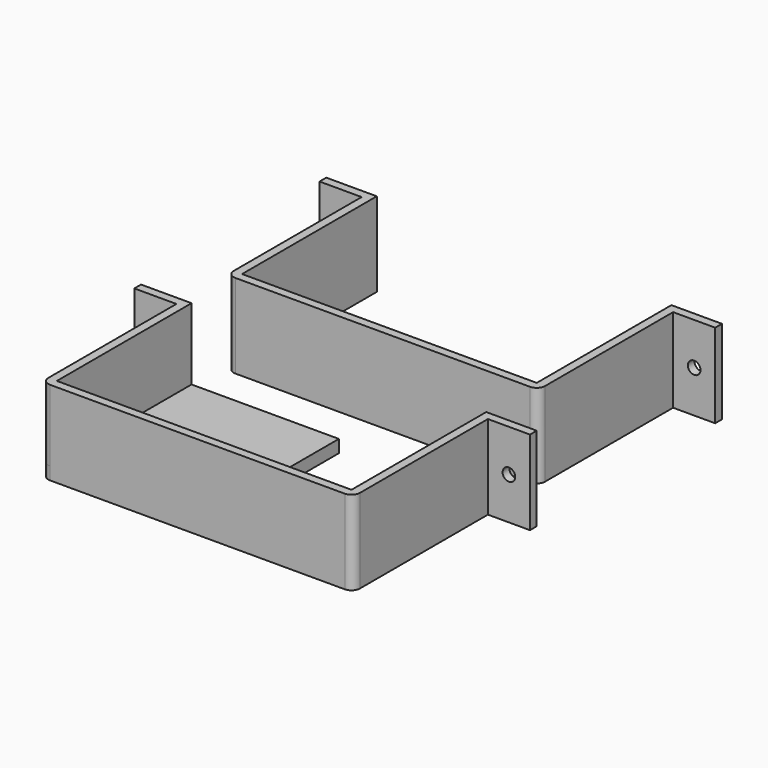
from build123d import *

# Parameters (mm, degrees)
F1_DEPTH = 20
F2_R     = 2
F4_D     = 3
F0_W     = 35
F0_H     = 40
F8_DEPTH = 3
F9_R     = 2


with BuildPart() as f1:
    # F0 (on Top) → F1 (new body)
    with BuildSketch(Plane.XY):
        Polygon((-15.9594300253, -31.1998534369), (-15.9594300253, 8.8001465631), (-27.9594300253, 8.8001465631), (-27.9594300253, 6.8001465631), (-17.9594300253, 6.8001465631), (-17.9594300253, -33.1998534369), (19.0405699747, -33.1998534369), (19.0405699747, -31.1998534369), align=None)
    extrude(amount=F1_DEPTH)

    # F2
    f2_edges = [f1.edges().sort_by_distance(p)[0] for p in [
        (-17.95943, -33.199853, 10),
    ]]
    fillet(f2_edges, radius=F2_R)

    # F4 (through all)
    with Locations(Plane.XZ.offset(-6.8001465631)):
        with Locations((-22.9594300253, 10)):
            Hole(F4_D / 2)

    # F5: F1 across face


with BuildPart() as f1_1:
    add(f1.part)
    add(f1.part.mirror(Plane(origin=(19.0405699747, -32.1998534369, 10), x_dir=(0, 1, 0), z_dir=(1, 0, 0))))


with BuildPart() as f6_1:
    # F6: copy of F1
    add(f1_1.part)


with BuildPart() as f6_1_1:
    # F7: moved
    add(f6_1.part.moved(Location((0, 55, 0))))


with BuildPart() as f1_2:
    add(f1_1.part)

    # F0 (on Top) → F8 (join)
    with BuildSketch(Plane.XY):
        with Locations((1.5405699747, -11.1998534369)):
            Rectangle(F0_W, F0_H)
        Polygon((-15.9594300253, -31.1998534369), (-15.9594300253, 8.8001465631), (-27.9594300253, 8.8001465631), (-27.9594300253, 6.8001465631), (-17.9594300253, 6.8001465631), (-17.9594300253, -33.1998534369), (19.0405699747, -33.1998534369), (19.0405699747, -31.1998534369), align=None)
    extrude(amount=F8_DEPTH)

    # F9
    f9_edges = [f1_2.edges().sort_by_distance(p)[0] for p in [
        (-17.95943, -33.199853, 1.5),
    ]]
    fillet(f9_edges, radius=F9_R)


solid = Compound([f6_1_1.part, f1_2.part])
